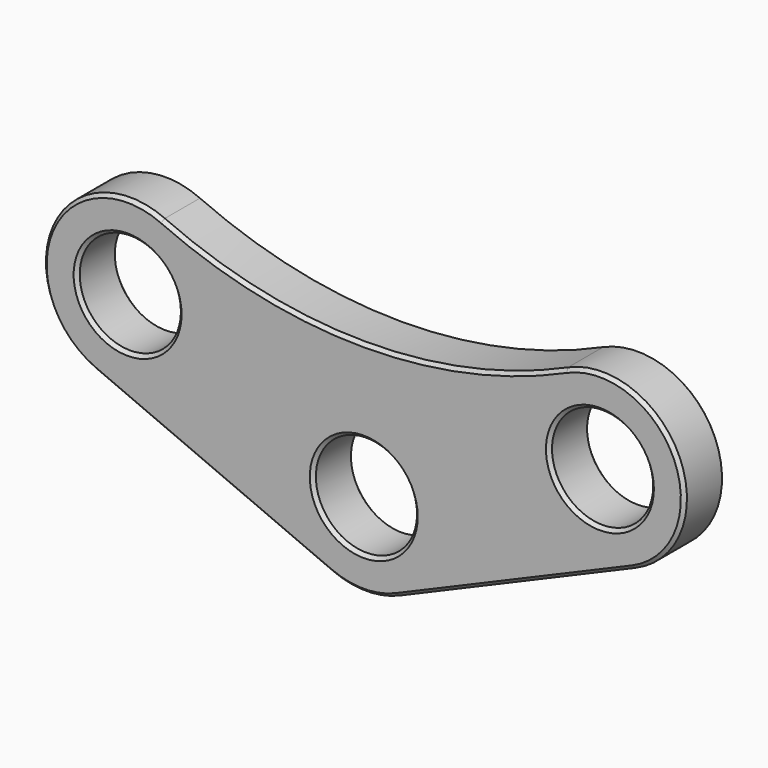
from build123d import *

# Parameters (mm, degrees)
F0_R     = 19.05
F1_DEPTH = 9.525
F2_SIZE  = 1.27


# Not quite as in the source:
# - a feature names something its author has since deleted; it is built from what else it names


with BuildPart() as f1:
    # F0 (on Front) → F1 (new body, symmetric)
    with BuildSketch(Plane.XZ):
        with BuildLine():
            Line((-101.4069377299, 8.9171452969), (-12.5069377299, -29.1828547031))
            ThreePointArc((-12.5069377299, -29.1828547031), (0, -31.75), (12.5069377299, -29.1828547031))
            Line((12.5069377299, -29.1828547031), (101.4069377299, 8.9171452969))
            ThreePointArc((101.4069377299, 8.9171452969), (117.9736119422, 50.8588239518), (75.8902439024, 67.062195122))
            ThreePointArc((75.8902439024, 67.062195122), (0, 50.8), (-75.8902439024, 67.062195122))
            ThreePointArc((-75.8902439024, 67.062195122), (-117.9736119422, 50.8588239518), (-101.4069377299, 8.9171452969))
        make_face()
        Circle(F0_R, mode=Mode.SUBTRACT)
        with Locations((-88.9, 38.1)):
            Circle(F0_R, mode=Mode.SUBTRACT)
        with Locations((88.9, 38.1)):
            Circle(F0_R, mode=Mode.SUBTRACT)
    extrude(amount=F1_DEPTH, both=True)

    # F2
    f2_edges = [f1.edges().sort_by_distance(p)[0] for p in [
        (-117.973612, -9.525, 50.858824),
        (-56.956938, -9.525, -10.132855),
        (0, -9.525, -31.75),
        (56.956938, -9.525, -10.132855),
        (117.973612, -9.525, 50.858824),
        (0, -9.525, 50.8),
        (-56.956938, 9.525, -10.132855),
        (0, 9.525, -31.75),
        (56.956938, 9.525, -10.132855),
        (117.973612, 9.525, 50.858824),
        (0, 9.525, 50.8),
        (-117.973612, 9.525, 50.858824),
        (-19.05, 9.525, 0),
        (-107.95, 9.525, 38.1),
        (69.85, 9.525, 38.1),
        (-19.05, -9.525, 0),
        (-107.95, -9.525, 38.1),
        (69.85, -9.525, 38.1),
    ]]
    chamfer(f2_edges, length=F2_SIZE)


solid = f1.part
